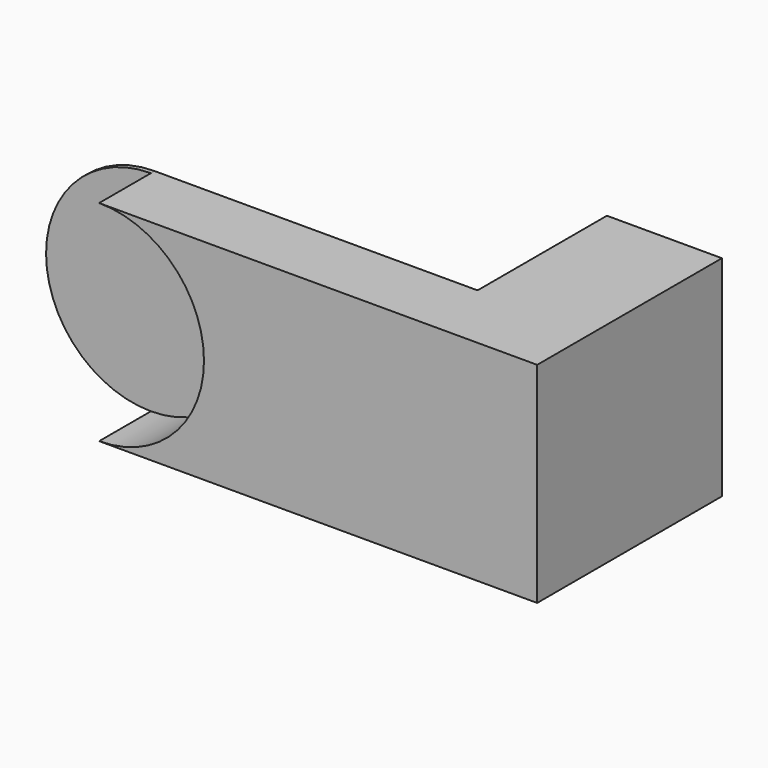
from build123d import *

# Parameters (mm, degrees)
F2_DEPTH = 15
F3_W     = 24.9072536826
F3_H     = 45.3870967031
F4_DEPTH = 50
F5_DEPTH = 1


# Not quite as in the source:
# - the program builds the solid bodies; features that only make, move or delete a surface that nothing else refers to are left out


with BuildPart() as f2:
    # F0 (on Front) → F2 (new body)
    with BuildSketch(Plane.XZ):
        with BuildLine():
            ThreePointArc((-58.766130358, 22.6935483515), (-42.7193684294, 16.0467619285), (-36.0725820065, 0))
            ThreePointArc((-36.0725820065, 0), (-42.7193684294, -16.0467619285), (-58.766130358, -22.6935483515))
            Line((-58.766130358, -22.6935483515), (36.0725782812, -22.6935483515))
            Line((36.0725782812, -22.6935483515), (36.0725782812, 22.6935483515))
            Line((36.0725782812, 22.6935483515), (-58.766130358, 22.6935483515))
        make_face()
    extrude(amount=F2_DEPTH)

    # F3 (on face) → F4 (join)
    with BuildSketch(Plane.XZ.offset(15)):
        with Locations((23.6189514399, 0)):
            Rectangle(F3_W, F3_H)
    extrude(amount=-F4_DEPTH)

    # F0 (on Front) → F5 (join)
    with BuildSketch(Plane.XZ):
        with BuildLine():
            ThreePointArc((-58.766130358, -22.6935483515), (-42.7193684294, -16.0467619285), (-36.0725820065, 0))
            ThreePointArc((-36.0725820065, 0), (-42.7193684294, 16.0467619285), (-58.766130358, 22.6935483515))
            Line((-58.766130358, 22.6935483515), (-58.766130358, -22.6935483515))
        make_face()
        with BuildLine():
            Line((-58.766130358, -22.6935483515), (-58.766130358, 22.6935483515))
            ThreePointArc((-58.766130358, 22.6935483515), (-81.4596787095, 0), (-58.766130358, -22.6935483515))
        make_face()
    extrude(amount=F5_DEPTH)


solid = f2.part
